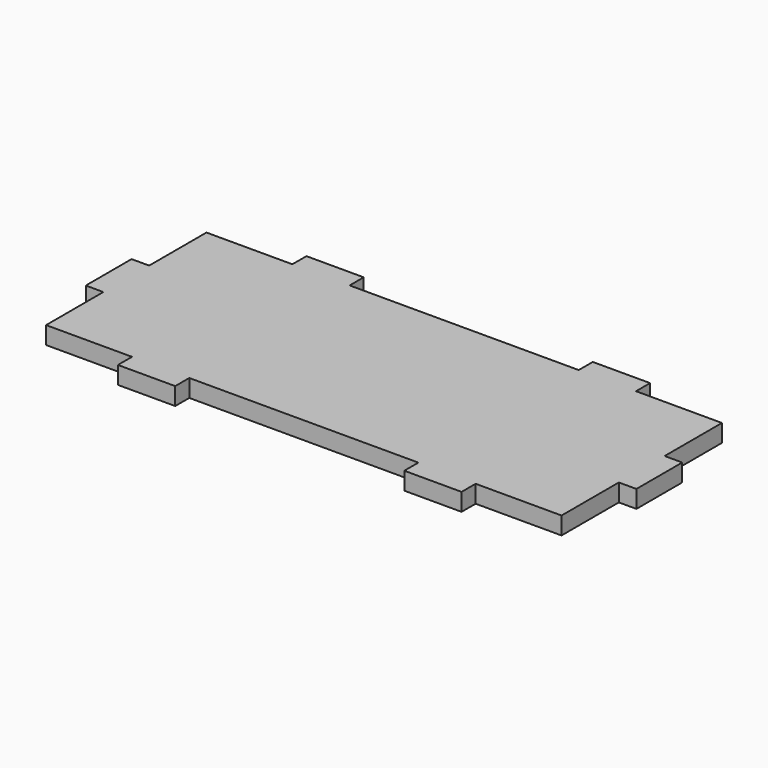
from build123d import *

# Parameters (mm, degrees)
F2_DEPTH = 6.14


# Not quite as in the source:
# - a feature names something its author has since deleted; it is built from what else it names


with BuildPart() as f2:
    # F1 (on Top) → F2 (new body)
    with BuildSketch(Plane.XY):
        Polygon((90, 10), (90, 35), (60, 35), (60, 41.14), (40, 41.14), (40, 35), (-40, 35), (-40, 41.14), (-60, 41.14), (-60, 35), (-90, 35), (-90, 10), (-96.14, 10), (-96.14, -10), (-90, -10), (-90, -35), (-60, -35), (-60, -41.14), (-40, -41.14), (-40, -35), (40, -35), (40, -41.14), (60, -41.14), (60, -35), (90, -35), (90, -10), (96.14, -10), (96.14, 10), align=None)
    extrude(amount=F2_DEPTH)


solid = f2.part
